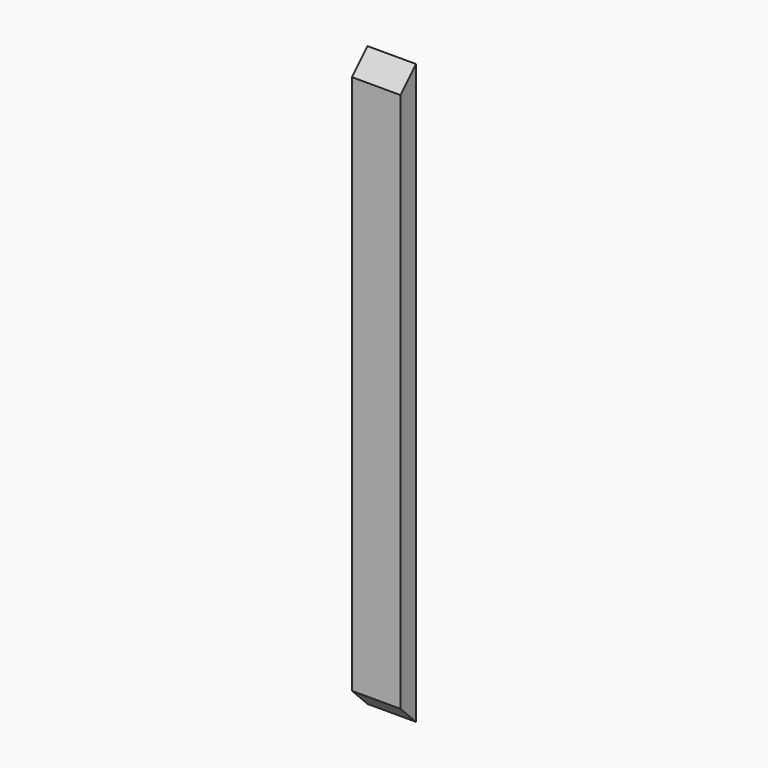
from build123d import *

# Parameters (mm, degrees)
F0_W     = 25
F0_H     = 298
F1_DEPTH = 10
F2_SIZE2 = 9.99999
F2_SIZE  = 9.99999


# Not quite as in the source:
# - a fillet or chamfer is up to 0.001 mm smaller than in the source, because OpenCascade refuses the exact size


with BuildPart() as f1:
    # F0 (on Front) → F1 (new body)
    with BuildSketch(Plane.XZ):
        Rectangle(F0_W, F0_H)
    extrude(amount=F1_DEPTH)

    # F2 (size 10 and 10 in the source; OpenCascade refuses exactly that, so slightly less here)
    f2_edges = [f1.edges().sort_by_distance(p)[0] for p in [
        (0, -10, 149),
        (0, -10, -149),
    ]]
    chamfer(f2_edges, length=F2_SIZE, length2=F2_SIZE2)


solid = f1.part
